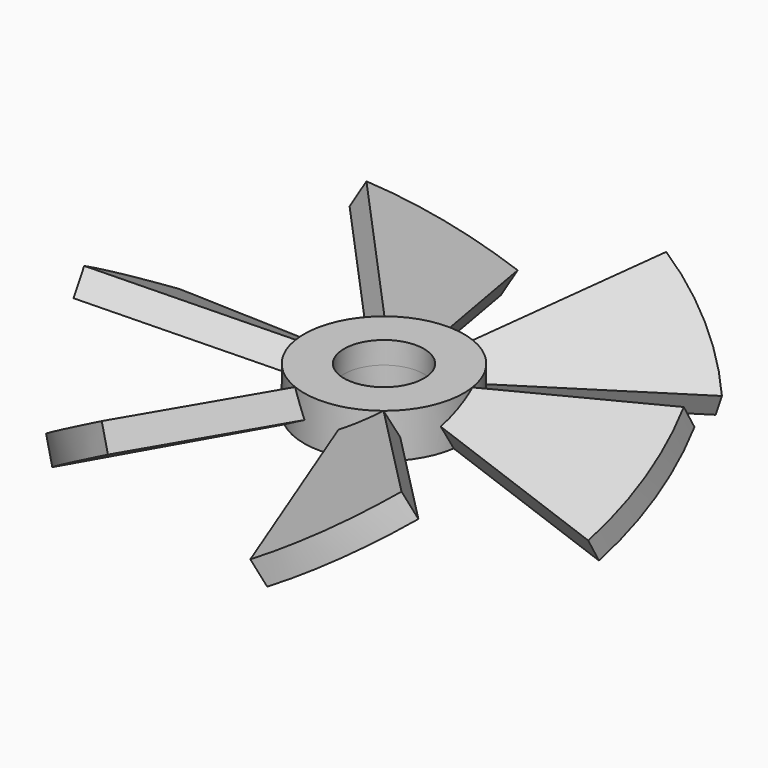
from build123d import *

# Parameters (mm, degrees)
F3_DEPTH      = 5
F3_DEPTH_BACK = 5
F5_COUNT      = 6
F6_R          = 30
F6_R_2        = 15
F8_DEPTH      = 8.3061646
F8_DEPTH_BACK = 8.3061646


# Not quite as in the source:
# - an extrude ends at something that could not be found from the text; its depth is read off the source's solid
# - a feature of the source that left no trace in its solid (it failed there, or was rolled back) is left out


with BuildPart() as f3:
    # F2 (on line) → F3 (new body, two sides)
    with BuildSketch(Plane(origin=(0, 0, 0), x_dir=(1, 0, 0), z_dir=(0, 0.5, -0.8660254038))) as f3_sk:
        with BuildLine():
            ThreePointArc((25, 0), (24.7861215343, -3.2631548055), (24.1481456572, -6.4704761276))
            Line((24.1481456572, -6.4704761276), (96.5925826289, -25.8819045103))
            ThreePointArc((96.5925826289, -25.8819045103), (99.1444861374, -13.052619222), (100, 0))
            ThreePointArc((100, 0), (99.1444861374, 13.052619222), (96.5925826289, 25.8819045103))
            Line((96.5925826289, 25.8819045103), (24.1481456572, 6.4704761276))
            ThreePointArc((24.1481456572, 6.4704761276), (24.7861215343, 3.2631548055), (25, 0))
        make_face()
    extrude(amount=F3_DEPTH)
    extrude(f3_sk.sketch, amount=-F3_DEPTH_BACK)


with BuildPart() as f5_1:
    # F5: instance of F3
    add(f3.part.rotate(Axis((0, 0, -4.0518213063), (0, 0, -1)), 1 * 360 / F5_COUNT))


with BuildPart() as f5_2:
    # F5: instance of F3
    add(f3.part.rotate(Axis((0, 0, -4.0518213063), (0, 0, -1)), 2 * 360 / F5_COUNT))


with BuildPart() as f5_3:
    # F5: instance of F3
    add(f3.part.rotate(Axis((0, 0, -4.0518213063), (0, 0, -1)), 3 * 360 / F5_COUNT))


with BuildPart() as f5_4:
    # F5: instance of F3
    add(f3.part.rotate(Axis((0, 0, -4.0518213063), (0, 0, -1)), 4 * 360 / F5_COUNT))


with BuildPart() as f5_5:
    # F5: instance of F3
    add(f3.part.rotate(Axis((0, 0, -4.0518213063), (0, 0, -1)), 5 * 360 / F5_COUNT))


with BuildPart() as f3_1:
    add(f3.part)

    add(f5_1.part)  # F8 merges F5_1

    add(f5_2.part)  # F8 merges F5_2

    add(f5_3.part)  # F8 merges F5_3

    add(f5_4.part)  # F8 merges F5_4

    add(f5_5.part)  # F8 merges F5_5
    # F6 (on Top) → F8 (join, two sides)
    with BuildSketch(Plane.XY) as f8_sk:
        Circle(F6_R)
        Circle(F6_R_2, mode=Mode.SUBTRACT)
    extrude(amount=F8_DEPTH)
    extrude(f8_sk.sketch, amount=-F8_DEPTH_BACK)


solid = f3_1.part
